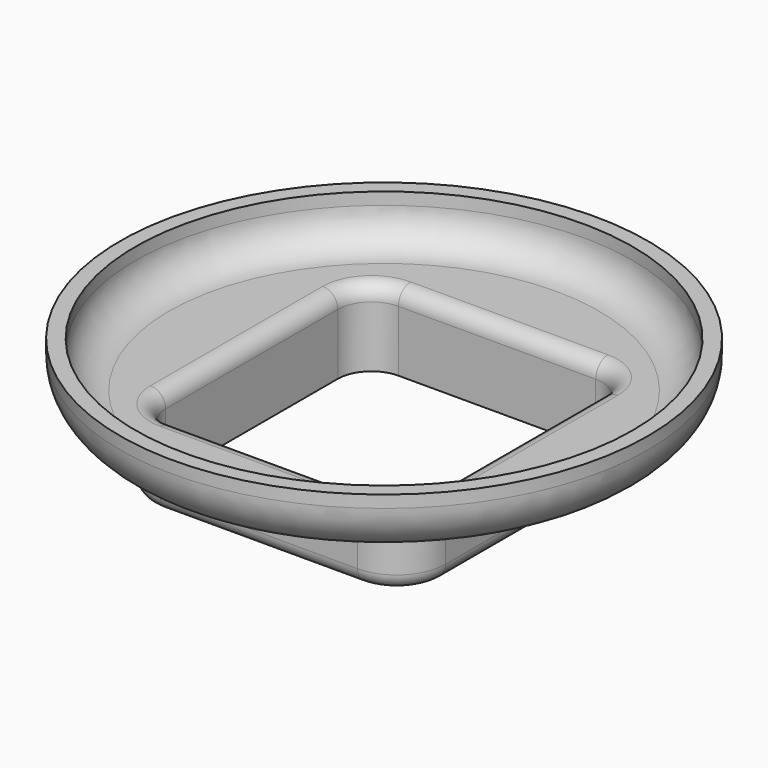
from build123d import *

# Parameters (mm, degrees)
F0_R     = 27.4307553129
F1_DEPTH = 6.35
F9_R     = 5.08
F2_T     = -1.5875
F3_W     = 30.6679024691
F3_H     = 32.5223739966
F4_DEPTH = 6.35
F5_R     = 5.08
F6_T     = -1.5875
F7_DEPTH = 6.351
F10_R    = 1.5875
F11_R    = 1.58749


# Not quite as in the source:
# - a fillet or chamfer is up to 0.001 mm smaller than in the source, because OpenCascade refuses the exact size


with BuildPart() as f1:
    # F0 (on Top) → F1 (new body)
    with BuildSketch(Plane.XY):
        Circle(F0_R)
    extrude(amount=F1_DEPTH)

    # F9
    f9_edges = [f1.edges().sort_by_distance(p)[0] for p in [
        (-27.430755, 0, 0),
    ]]
    fillet(f9_edges, radius=F9_R)

    # F2
    f2_openings = [f1.faces().sort_by_distance(p)[0] for p in [
        (0, 0, 6.35),
    ]]
    offset(amount=F2_T, openings=f2_openings)

    # F3 (on face) → F4 (join)
    with BuildSketch(Plane(origin=(0, 0, 0), x_dir=(1, 0, 0), z_dir=(0, 0, -1))):
        Rectangle(F3_W, F3_H)
    extrude(amount=F4_DEPTH)

    # F5
    f5_edges = [f1.edges().sort_by_distance(p)[0] for p in [
        (-15.333951, 16.261187, -3.175),
        (-15.333951, -16.261187, -3.175),
        (15.333951, -16.261187, -3.175),
        (15.333951, 16.261187, -3.175),
    ]]
    fillet(f5_edges, radius=F5_R)

    # F6
    f6_openings = [f1.faces().sort_by_distance(p)[0] for p in [
        (0, 0, -6.35),
    ]]
    offset(amount=F6_T, openings=f6_openings, kind=Kind.INTERSECTION)

    # F7 (cut, through all): a face of the model
    f7_faces = [f1.faces().sort_by_distance(p)[0] for p in [
        (0, 0, 0),
    ]]
    extrude(f7_faces, amount=-F7_DEPTH, mode=Mode.SUBTRACT)

    # F10
    f10_edges = [f1.edges().sort_by_distance(p)[0] for p in [
        (13.746451, 0, 1.5875),
    ]]
    fillet(f10_edges, radius=F10_R)

    # F11 (radius 1.5875 in the source; OpenCascade refuses exactly that, so slightly less here)
    f11_edges = [f1.edges().sort_by_distance(p)[0] for p in [
        (15.333951, 0, 0),
        (15.333951, 11.181187, -3.175),
        (15.333951, -11.181187, -3.175),
        (15.333951, 0, -6.35),
    ]]
    fillet(f11_edges, radius=F11_R)


solid = f1.part
